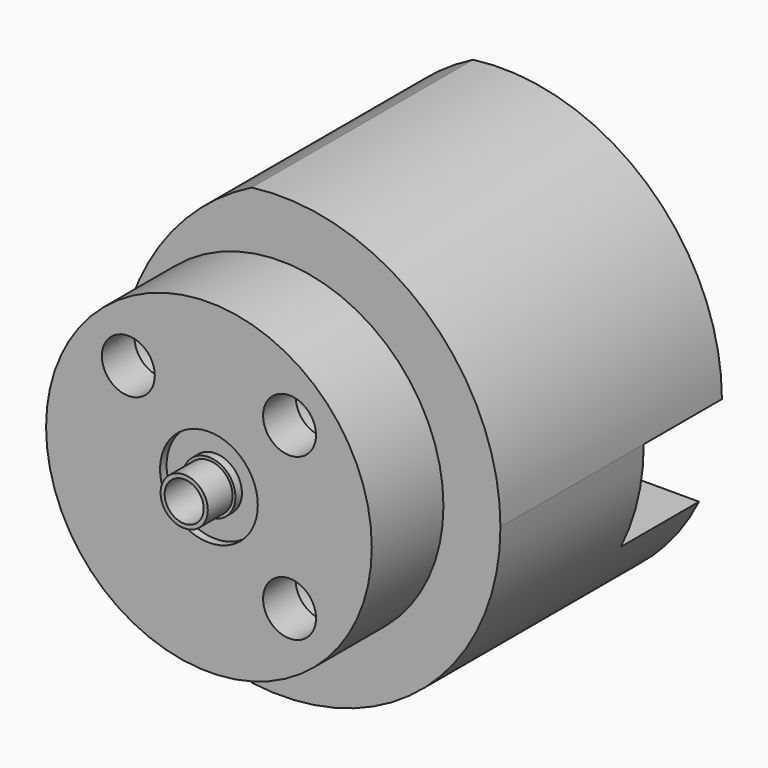
from build123d import *

# Parameters (mm, degrees)
F0_R      = 27
F1_DEPTH  = 45
F2_R      = 41.8433440982
F2_R_2    = 20
F3_DEPTH  = 11
F5_D      = 6.5
F5_DEPTH  = 50
F5_TIP    = 1.9527970118
F6_R      = 5.25
F7_DEPTH  = 40
F8_R      = 2.9
F9_DEPTH  = 3.8
F10_R     = 2.4
F11_DEPTH = 8
F12_R     = 6
F12_R_2   = 3.2524774455
F13_DEPTH = 1
F15_DEPTH = 12
F16_R     = 45.2689658455
F16_R_2   = 30
F17_DEPTH = 53.4


# Not quite as in the source:
# - a feature names something its author has since deleted; it is built from what else it names


with BuildPart() as f1:
    # F0 (on Front) → F1 (new body)
    with BuildSketch(Plane.XZ):
        Circle(F0_R)
    extrude(amount=F1_DEPTH)

    # F2 (on face) → F3 (cut)
    with BuildSketch(Plane.XZ.offset(45)):
        Circle(F2_R)
        Circle(F2_R_2, mode=Mode.SUBTRACT)
    extrude(amount=-F3_DEPTH, mode=Mode.SUBTRACT)

    # F5
    with Locations(Plane(origin=(0, 0, 0), x_dir=(-1, 0, 0), z_dir=(0, 1, 0))):
        with Locations((-9.8994949366, 9.8994949366), (9.8994949366, 9.8994949366), (-9.8994949366, -9.8994949366)):
            Hole(F5_D / 2, depth=F5_DEPTH)
            with Locations((0, 0, -(F5_DEPTH + F5_TIP / 2))):  # 118° drill point
                Cone(0, F5_D / 2, F5_TIP, mode=Mode.SUBTRACT)

    # F6 (on face) → F7 (cut)
    with BuildSketch(Plane(origin=(0, 0, 0), x_dir=(-1, 0, 0), z_dir=(0, 1, 0))):
        with Locations((-9.8994949366, -9.8994949366)):
            Circle(F6_R)
        with Locations((9.8994949366, 9.8994949366)):
            Circle(F6_R)
        with Locations((-9.8994949366, 9.8994949366)):
            Circle(F6_R)
    extrude(amount=-F7_DEPTH, mode=Mode.SUBTRACT)

    # F8 (on face) → F9 (join)
    with BuildSketch(Plane.XZ.offset(45)):
        Circle(F8_R)
    extrude(amount=F9_DEPTH)

    # F10 (on face) → F11 (cut)
    with BuildSketch(Plane.XZ.offset(48.8)):
        Circle(F10_R)
    extrude(amount=-F11_DEPTH, mode=Mode.SUBTRACT)

    # F12 (on face) → F13 (cut)
    with BuildSketch(Plane.XZ.offset(45)):
        Circle(F12_R)
        Circle(F12_R_2, mode=Mode.SUBTRACT)
    extrude(amount=-F13_DEPTH, mode=Mode.SUBTRACT)

    # F14 (on face) → F15 (cut)
    with BuildSketch(Plane(origin=(0, 0, 0), x_dir=(-1, 0, 0), z_dir=(0, 1, 0))):
        Polygon((39.7908514319, 0), (0, 0), (-37.339406552, 0), (-37.339406552, -12), (41.6823292512, -12), align=None)
    extrude(amount=-F15_DEPTH, mode=Mode.SUBTRACT)

    # F16 (on face) → F17 (cut)
    with BuildSketch(Plane(origin=(0, 0, 0), x_dir=(-1, 0, 0), z_dir=(0, 1, 0))):
        with Locations((-10, 0)):
            Circle(F16_R)
        with Locations((-10, 0)):
            Circle(F16_R_2, mode=Mode.SUBTRACT)
    extrude(amount=-F17_DEPTH, mode=Mode.SUBTRACT)


solid = f1.part
